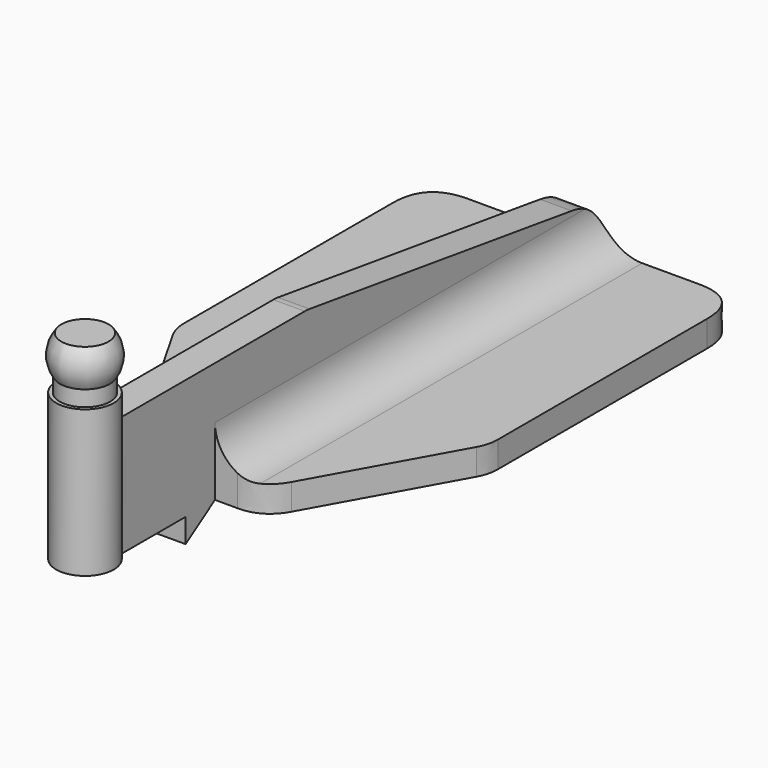
from build123d import *
from build123d import SkipClean  # not in build123d's __all__

# Parameters (mm, degrees)
F1_DEPTH      = 3.175
F2_W          = 1.905
F2_H          = 58.42
F3_DEPTH      = 11.43
F4_DEPTH      = 20.955
F5_DEPTH      = 3.175
F7_DEPTH      = 25.4
F8_DEPTH      = 3.81
F4_FACE_R     = 3.4925
F9_DEPTH      = 6.35
F10_W         = 0.508
F10_H         = 0.508
F11_DEPTH     = 6.35
F14_T1_DEPTH  = 25.8393032031
F14_T3_DEPTH  = 5.6151224214
F14_T5_DEPTH  = 28.575
F14_T7_DEPTH  = 9.7559624537
F14_T9_DEPTH  = 18.1215030756
F14_T11_DEPTH = 9.900818989
F14_T13_DEPTH = 17.9395791643
F15_R         = 5.08


# Not quite as in the source:
# - a fillet or chamfer that OpenCascade refuses, or shapes differently, is made with other operations: its cross-section is extruded or revolved along the edge and cut away or added
# - after a boolean that leaves OpenCascade's solid faulty, fix() repairs it


with BuildPart() as f1:
    # F0 (on Top) → F1 (new body)
    with BuildSketch(Plane.XY):
        Polygon((-19.05, 6.2771309167), (-7.4772434087, -14.0428690833), (0, -14.0428690833), (0, 44.3771309167), (-19.05, 44.3771309167), align=None)
        Polygon((0, 44.3771309167), (0, -14.0428690833), (7.7627565913, -14.0428690833), (19.05, 6.2771309167), (19.05, 44.3771309167), align=None)
    extrude(amount=F1_DEPTH)

    # F2 (on face) → F3 (join)
    with BuildSketch(Plane.XY.offset(3.175)):
        with Locations((-0.8097434087, 15.1671309167)):
            Rectangle(F2_W, F2_H)
        with Locations((1.0952565913, 15.1671309167)):
            Rectangle(F2_W, F2_H)
        with BuildLine():
            Line((2.0477565913, -14.0428690833), (0.1427565913, -14.0428690833))
            Line((0.1427565913, -14.0428690833), (-1.7622434087, -14.0428690833))
            Line((-1.7622434087, -14.0428690833), (-1.7622434087, -28.1725657124))
            ThreePointArc((-1.7622434087, -28.1725657124), (0.1704115334, -27.6995290541), (2.0477565913, -28.3586909))
            Line((2.0477565913, -28.3586909), (2.0477565913, -14.0428690833))
        make_face()
    extrude(amount=F3_DEPTH)

    # F2 (on face) → F4 (join)
    with BuildSketch(Plane.XY.offset(3.175)):
        with BuildLine():
            ThreePointArc((2.0477565913, -28.3586909), (0.1704115334, -27.6995290541), (-1.7622434087, -28.1725657124))
            ThreePointArc((-1.7622434087, -28.1725657124), (-1.7382349014, -34.217076187), (3.4925, -31.1878690833))
            ThreePointArc((3.4925, -31.1878690833), (3.1104136497, -29.5995104407), (2.0477565913, -28.3586909))
        make_face()
    extrude(amount=F4_DEPTH)

    # F2 (on face) → F5 (join)
    with BuildSketch(Plane.XY.offset(3.175)):
        with BuildLine():
            Line((2.0477565913, 44.3771309167), (0.1427565913, 44.3771309167))
            Line((0.1427565913, 44.3771309167), (-1.7622434087, 44.3771309167))
            Line((-1.7622434087, 44.3771309167), (-1.7622434087, -28.1725657124))
            ThreePointArc((-1.7622434087, -28.1725657124), (0.1704115334, -27.6995290541), (2.0477565913, -28.3586909))
            Line((2.0477565913, -28.3586909), (2.0477565913, 44.3771309167))
        make_face()
        with BuildLine():
            ThreePointArc((2.0477565913, -28.3586909), (0.1704115334, -27.6995290541), (-1.7622434087, -28.1725657124))
            ThreePointArc((-1.7622434087, -28.1725657124), (-1.7382349014, -34.217076187), (3.4925, -31.1878690833))
            ThreePointArc((3.4925, -31.1878690833), (3.1104136497, -29.5995104407), (2.0477565913, -28.3586909))
        make_face()
    with SkipClean():  # cleaning this boolean's faces spoils the solid; the shape is the same uncleaned
        extrude(amount=-F5_DEPTH)

    # F6 (on face) → F7 (cut)
    with BuildSketch(Plane.YZ.offset(2.0477565913)):
        Polygon((44.3771309167, 8.255), (44.3771309167, 14.605), (-0.0728690833, 14.605), align=None)
    extrude(amount=-F7_DEPTH, mode=Mode.SUBTRACT)

    add(f1.part.fix(), mode=Mode.REPLACE)

    # F6 (on face) → F8 (join)
    with BuildSketch(Plane.YZ.offset(2.0477565913)):
        Polygon((-18.4878690833, -2.921), (-14.0428690833, 0), (-18.4878690833, 0), align=None)
    extrude(amount=-F8_DEPTH)

    add(f1.part.fix(), mode=Mode.REPLACE)

    # F4_face (on face) → F9 (cut)
    with BuildSketch(Plane(origin=(0, -31.1878690833, 24.13), x_dir=(1, 0, 0), z_dir=(0, 0, 1))):
        Circle(F4_FACE_R)
    extrude(amount=-F9_DEPTH, mode=Mode.SUBTRACT)

    # F10 (on face) → F11 (join)
    with BuildSketch(Plane.XY.offset(17.78)):
        with Locations((0.254, -30.9338690833)):
            Rectangle(F10_W, F10_H)
    extrude(amount=F11_DEPTH)

    # F12 (on face) → F13 (revolve)
    with BuildSketch(Plane(origin=(0, 0, 0), x_dir=(0, -1, 0), z_dir=(-1, 0, 0))):
        with BuildLine():
            Line((31.1878690833, 24.13), (31.1878690833, 17.78))
            Line((31.1878690833, 17.78), (34.2358690833, 17.78))
            Line((34.2358690833, 17.78), (34.2358690833, 19.685))
            ThreePointArc((34.2358690833, 19.685), (34.8876462819, 21.9395154514), (34.0453690833, 24.13))
            Line((34.0453690833, 24.13), (31.1878690833, 24.13))
        make_face()
    revolve(axis=Axis((0, -31.1878690833, 20.955), (0, 0, 1)))

    # F14: fillet of radius 5.08 on 8 edges, made by hand

    # F14_s2 → F14_t1 (cut)
    with BuildSketch(Plane.YZ.offset(-12.7768950102)):
        with BuildLine():
            add(Edge.make_bspline(
                [(40.0155514064, 8.8780827872), (44.3771309167, 8.255), (44.3771309167, 3.8491393594)],
                knots=[0, 0, 0, 1, 1, 1], degree=2, weights=[1, 1, 1]))
            Line((44.3771309167, 3.8491393594), (44.3771309167, 8.255))
            Line((44.3771309167, 8.255), (40.0155514064, 8.8780827872))
        make_face()
    extrude(amount=F14_T1_DEPTH, mode=Mode.SUBTRACT)

    # F14_s4 → F14_t3 (cut)
    with BuildSketch(Plane.YZ.offset(-2.6648046194)):
        with BuildLine():
            add(Edge.make_bspline(
                [(-0.4338935676, 14.605), (-0.0728690833, 14.605), (0.2845269221, 14.5539434278)],
                knots=[0, 0, 0, 1, 1, 1], degree=2, weights=[1, 1, 1]))
            Line((0.2845269221, 14.5539434278), (-0.0728690833, 14.605))
            Line((-0.0728690833, 14.605), (-0.4338935676, 14.605))
        make_face()
    extrude(amount=F14_T3_DEPTH, mode=Mode.SUBTRACT)

    # F14_s6 → F14_t5 (cut)
    with BuildSketch(Plane.XY.offset(-12.7)):
        with BuildLine():
            add(Edge.make_bspline(
                [(13.97, 44.3771309167), (19.05, 44.3771309167), (19.05, 39.2971309167)],
                knots=[0, 0, 0, 1, 1, 1], degree=2, weights=[1, 1, 1]))
            Line((19.05, 39.2971309167), (19.05, 44.3771309167))
            Line((19.05, 44.3771309167), (13.97, 44.3771309167))
        make_face()
        with BuildLine():
            add(Edge.make_bspline(
                [(-13.97, 44.3771309167), (-19.05, 44.3771309167), (-19.05, 39.2971309167)],
                knots=[0, 0, 0, 1, 1, 1], degree=2, weights=[1, 1, 1]))
            Line((-19.05, 39.2971309167), (-19.05, 44.3771309167))
            Line((-19.05, 44.3771309167), (-13.97, 44.3771309167))
        make_face()
    extrude(amount=F14_T5_DEPTH, mode=Mode.SUBTRACT)

    # F14_s8 → F14_t7 (cut)
    with BuildSketch(Plane.XY.offset(-3.2904812268)):
        with BuildLine():
            add(Edge.make_bspline(
                [(19.05, 7.5933234075), (19.05, 6.2771309167), (18.4108716207, 5.1265321215)],
                knots=[0, 0, 0, 1, 1, 1], degree=2, weights=[1, 1, 1]))
            Line((18.4108716207, 5.1265321215), (19.05, 6.2771309167))
            Line((19.05, 6.2771309167), (19.05, 7.5933234075))
        make_face()
    extrude(amount=F14_T7_DEPTH, mode=Mode.SUBTRACT)

    # F14_s10 → F14_t9 (cut)
    with BuildSketch(Plane.XY.offset(-7.4732515378)):
        with BuildLine():
            add(Edge.make_bspline(
                [(4.7734559762, -14.0428690833), (7.7627565913, -14.0428690833), (9.2143275969, -11.4296603692)],
                knots=[0, 0, 0, 1, 1, 1], degree=2, weights=[1, 1, 1]))
            Line((9.2143275969, -11.4296603692), (7.7627565913, -14.0428690833))
            Line((7.7627565913, -14.0428690833), (4.7734559762, -14.0428690833))
        make_face()
    extrude(amount=F14_T9_DEPTH, mode=Mode.SUBTRACT)

    # F14_s12 → F14_t11 (cut)
    with BuildSketch(Plane.XY.offset(-3.3629094945)):
        with BuildLine():
            add(Edge.make_bspline(
                [(-19.05, 7.6222947145), (-19.05, 6.2771309167), (-18.3842895287, 5.1082446043)],
                knots=[0, 0, 0, 1, 1, 1], degree=2, weights=[1, 1, 1]))
            Line((-18.3842895287, 5.1082446043), (-19.05, 6.2771309167))
            Line((-19.05, 6.2771309167), (-19.05, 7.6222947145))
        make_face()
    extrude(amount=F14_T11_DEPTH, mode=Mode.SUBTRACT)

    # F14_s14 → F14_t13 (cut)
    with BuildSketch(Plane.XY.offset(-7.3822895821)):
        with BuildLine():
            add(Edge.make_bspline(
                [(-4.5243275759, -14.0428690833), (-7.4772434087, -14.0428690833), (-8.9386171046, -11.4769191935)],
                knots=[0, 0, 0, 1, 1, 1], degree=2, weights=[1, 1, 1]))
            Line((-8.9386171046, -11.4769191935), (-7.4772434087, -14.0428690833))
            Line((-7.4772434087, -14.0428690833), (-4.5243275759, -14.0428690833))
        make_face()
    extrude(amount=F14_T13_DEPTH, mode=Mode.SUBTRACT)

    # F15 (call 1 of 2: OpenCascade refuses the feature's edges together)
    f15_edges = [f1.edges().sort_by_distance(p)[0] for p in [
        (-1.762243, 15.167131, 3.175),
    ]]
    fillet(f15_edges, radius=F15_R)

    # F15#2 (call 2 of 2)
    f15_2_edges = [f1.edges().sort_by_distance(p)[0] for p in [
        (2.047757, 15.167131, 3.175),
    ]]
    fillet(f15_2_edges, radius=F15_R)


solid = f1.part
